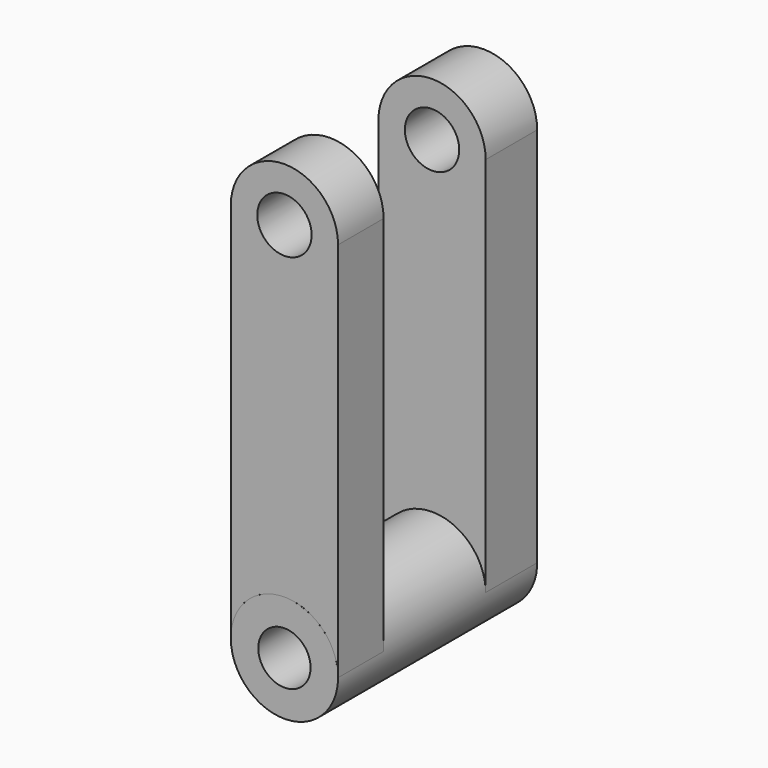
from build123d import *

# Parameters (mm, degrees)
F0_R          = 5.4593234286
F4_DEPTH      = 50
F5_W          = 25.6320154294
F5_H          = 97.1445217729
F6_DEPTH      = 25
F6_DEPTH_BACK = 25
F0_R_2        = 5.255163488
F7_DEPTH      = 50


# Not quite as in the source:
# - a feature of the source that left no trace in its solid (it failed there, or was rolled back) is left out


with BuildPart() as f4:
    # F0 (on Front) → F4 (new body)
    with BuildSketch(Plane.XZ):
        with BuildLine():
            Line((-10.0398408249, 48.2121519744), (-10.0398408249, -28.3416360617))
            ThreePointArc((-10.0398408249, -28.3416360617), (0.7320712321, -17.5697240047), (11.503983289, -28.3416360617))
            Line((11.503983289, -28.3416360617), (11.503983289, 48.2121519744))
            ThreePointArc((11.503983289, 48.2121519744), (0.7320712321, 58.9840640314), (-10.0398408249, 48.2121519744))
        make_face()
        with Locations((0.7320712321, 48.2121519744)):
            Circle(F0_R, mode=Mode.SUBTRACT)
    extrude(amount=F4_DEPTH)

    # F5 (on Right) → F6 (cut, two sides)
    with BuildSketch(Plane.YZ) as f6_sk:
        with Locations((-25.7514272816, 18.2514749467)):
            Rectangle(F5_W, F5_H)
    extrude(amount=F6_DEPTH, mode=Mode.SUBTRACT)
    extrude(f6_sk.sketch, amount=-F6_DEPTH_BACK, mode=Mode.SUBTRACT)


with BuildPart() as f7:
    # F0 (on Front) → F7 (new body)
    with BuildSketch(Plane.XZ):
        with BuildLine():
            ThreePointArc((11.503983289, -28.3416360617), (0.7320712321, -17.5697240047), (-10.0398408249, -28.3416360617))
            ThreePointArc((-10.0398408249, -28.3416360617), (0.7320712321, -39.1135481186), (11.503983289, -28.3416360617))
        make_face()
        with Locations((0.7320712321, -28.3416360617)):
            Circle(F0_R_2, mode=Mode.SUBTRACT)
    extrude(amount=F7_DEPTH)


solid = Compound([f4.part, f7.part])
